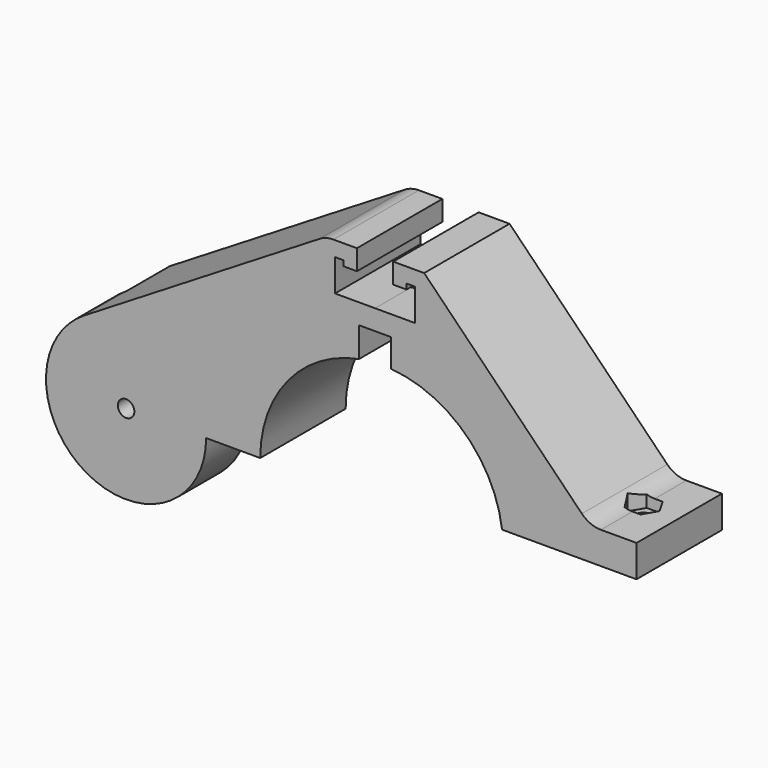
from build123d import *

# Parameters (mm, degrees)
F1_DEPTH  = 10
F0_R      = 1.55
F2_DEPTH  = 10
F4_DEPTH  = 50
F6_DEPTH  = 4
F7_R      = 1.5
F8_DEPTH  = 5
F9_R      = 1.5
F10_DEPTH = 25
F11_R     = 1.5
F12_DEPTH = 25


# Not quite as in the source:
# - ends of sketch curves that miss each other by under 0.0002 mm in the source are joined


with BuildPart() as f1:
    # F0 (on Front) → F1 (new body, symmetric)
    with BuildSketch(Plane.XZ):
        with BuildLine():
            ThreePointArc((-22.75, 0), (-1.4668388401, 22.702662483), (22.560846929, 2.9275733717))
            Line((22.560846929, 2.9275733717), (25.5830376256, 2.9275733717))
            Line((25.5830376256, 2.9275733717), (47.75, 2.9275733717))
            Line((47.75, 2.9275733717), (47.75, 8.9275733717))
            Line((47.75, 8.9275733717), (41.0830374761, 8.9275733717))
            ThreePointArc((41.0830374761, 8.9275733717), (39.1491782862, 9.316696163), (37.5163225707, 10.4234979182))
            Line((37.5163225707, 10.4234979182), (7.964999938, 40.503085047))
            Line((7.964999938, 40.503085047), (2.164999938, 40.503085047))
            Line((2.164999938, 40.503085047), (2.164999938, 36.703085047))
            Line((2.164999938, 36.703085047), (4.664999938, 36.703085047))
            Line((4.664999938, 36.703085047), (4.664999938, 37.703085047))
            Line((4.664999938, 37.703085047), (6.264999938, 37.703085047))
            Line((6.264999938, 37.703085047), (6.264999938, 31.703085047))
            Line((6.264999938, 31.703085047), (-1.235000062, 31.703085047))
            Line((-1.235000062, 31.703085047), (-8.735000062, 31.7030854494))
            Line((-8.735000062, 31.7030854494), (-8.735000062, 37.7030854494))
            Line((-8.735000062, 37.7030854494), (-7.135000062, 37.7030854494))
            Line((-7.135000062, 37.7030854494), (-7.135000062, 36.7030854494))
            Line((-7.135000062, 36.7030854494), (-4.635000062, 36.7030854494))
            Line((-4.635000062, 36.7030854494), (-4.635000062, 40.5030854494))
            Line((-4.635000062, 40.5030854494), (-9.0264711097, 40.5030854494))
            ThreePointArc((-9.0264711097, 40.5030854494), (-10.3822316524, 40.3157680019), (-11.6364091533, 39.7678507898))
            Line((-11.6364091533, 39.7678507898), (-55.7125058122, 12.7942960211))
            ThreePointArc((-55.7125058122, 12.7942960211), (-40.5494526959, 13.0852438258), (-32.8826916814, 0))
            Line((-32.8826916814, 0), (-25.75, 0))
            Line((-25.75, 0), (-22.75, 0))
        make_face()
    extrude(amount=F1_DEPTH, both=True)

    # F0 (on Front) → F2 (join)
    with BuildSketch(Plane.XZ):
        with BuildLine():
            ThreePointArc((-55.7125058122, 12.7942960211), (-55.2159306669, -13.0852438258), (-32.8826916814, 0))
            ThreePointArc((-32.8826916814, 0), (-40.5494526959, 13.0852438258), (-55.7125058122, 12.7942960211))
        make_face()
        with Locations((-47.8826916814, 0)):
            Circle(F0_R, mode=Mode.SUBTRACT)
    extrude(amount=F2_DEPTH)

    # F3 (on face) → F4 (cut)
    with BuildSketch(Plane(origin=(0, 0, 2.9275733717), x_dir=(1, 0, 0), z_dir=(0, 0, -1))):
        Polygon((42.583, -2.5980762114), (44.083, 0), (42.583, 2.5980762114), (39.583, 2.5980762114), (38.083, 0), (39.583, -2.5980762114), align=None)
    extrude(amount=-F4_DEPTH, mode=Mode.SUBTRACT)

    # F5 (on face) → F6 (join)
    with BuildSketch(Plane(origin=(0, 0, 2.9275733717), x_dir=(1, 0, 0), z_dir=(0, 0, -1))):
        Polygon((42.583, 2.5980762114), (39.583, 2.5980762114), (38.083, 0), (39.583, -2.5980762114), (42.583, -2.5980762114), (44.083, 0), align=None)
    extrude(amount=-F6_DEPTH)

    # F7 (on face) → F8 (cut)
    with BuildSketch(Plane.XY.offset(6.9275733717)):
        with Locations((41.083, 0)):
            Circle(F7_R)
    extrude(amount=-F8_DEPTH, mode=Mode.SUBTRACT)

    # F9 (on face) → F10 (cut)
    with BuildSketch(Plane(origin=(0, 0, 2.9275733717), x_dir=(1, 0, 0), z_dir=(0, 0, -1))):
        Polygon((-4.235000062, 10), (-4.235000062, -10), (-1.235000062, -10), (1.764999938, -10), (1.764999938, 10), align=None)
        with Locations((-1.235000062, 0)):
            Circle(F9_R, mode=Mode.SUBTRACT)
    extrude(amount=-F10_DEPTH, mode=Mode.SUBTRACT)

    # F11 (on face) → F12 (cut)
    with BuildSketch(Plane.XY.offset(31.703085047)):
        with Locations((-1.235000062, 0)):
            Circle(F11_R)
    extrude(amount=-F12_DEPTH, mode=Mode.SUBTRACT)


solid = f1.part
